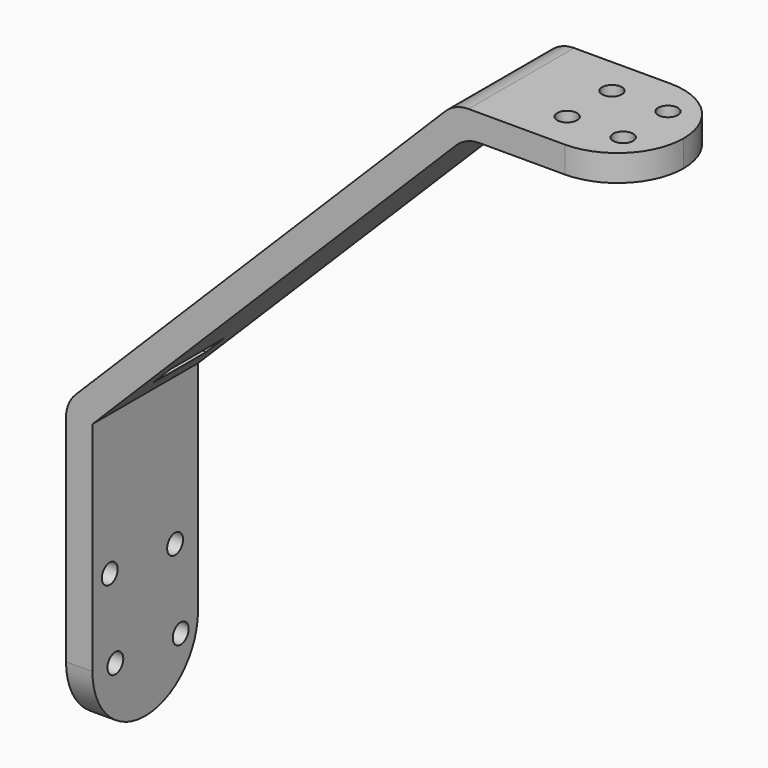
from build123d import *

# Parameters (mm, degrees)
F1_DEPTH = 20
F3_R     = 9.99999
F4_D     = 3
F5_R     = 5
F7_D     = 3
F8_W     = 4
F8_H     = 10
F9_DEPTH = 25


# Not quite as in the source:
# - a fillet or chamfer is up to 0.001 mm smaller than in the source, because OpenCascade refuses the exact size


with BuildPart() as f1:
    # F0 (on Front) → F1 (new body)
    with BuildSketch(Plane.XZ):
        Polygon((-4, 0), (0, 0), (0, 43), (56.5685424949, 99.5685424949), (81.5685424949, 99.5685424949), (81.5685424949, 103.5685424949), (54.9116882454, 103.5685424949), (-4, 44.6568542495), align=None)
    extrude(amount=F1_DEPTH)

    # F3 (radius 10 in the source; OpenCascade refuses exactly that, so slightly less here)
    f3_edges = [f1.edges().sort_by_distance(p)[0] for p in [
        (-2, -20, 0),
        (-2, 0, 0),
        (81.568542, 0, 101.568542),
        (81.568542, -20, 101.568542),
    ]]
    fillet(f3_edges, radius=F3_R)

    # F4 (through all)
    with Locations(Plane(origin=(0, 0, 99.5685424949), x_dir=(1, 0, 0), z_dir=(0, 0, -1))):
        with Locations((75.811183182, 14.2426406871), (67.3259018078, 14.2426406871), (67.3259018078, 5.7573593129), (75.811183182, 5.7573593129)):
            Hole(F4_D / 2)

    # F5
    f5_edges = [f1.edges().sort_by_distance(p)[0] for p in [
        (54.911688, -10, 103.568542),
        (56.568542, -10, 99.568542),
        (-4, -10, 44.656854),
    ]]
    fillet(f5_edges, radius=F5_R)

    # F7 (through all)
    with Locations(Plane.YZ):
        with Locations((-4.3431457505, 20.6568542495), (-16.7175144213, 21.7175144213), (-15.6568542495, 9.3431457505), (-3.2824855787, 8.2824855787)):
            Hole(F7_D / 2)

    # F8 (on face) → F9 (cut)
    with BuildSketch(Plane(origin=(-21.5, 0, 21.5), x_dir=(0.7071067812, 0, 0.7071067812), z_dir=(0.7071067812, 0, -0.7071067812))):
        with Locations((39.5918783247, 10)):
            Rectangle(F8_W, F8_H)
    extrude(amount=-F9_DEPTH, mode=Mode.SUBTRACT)


solid = f1.part
